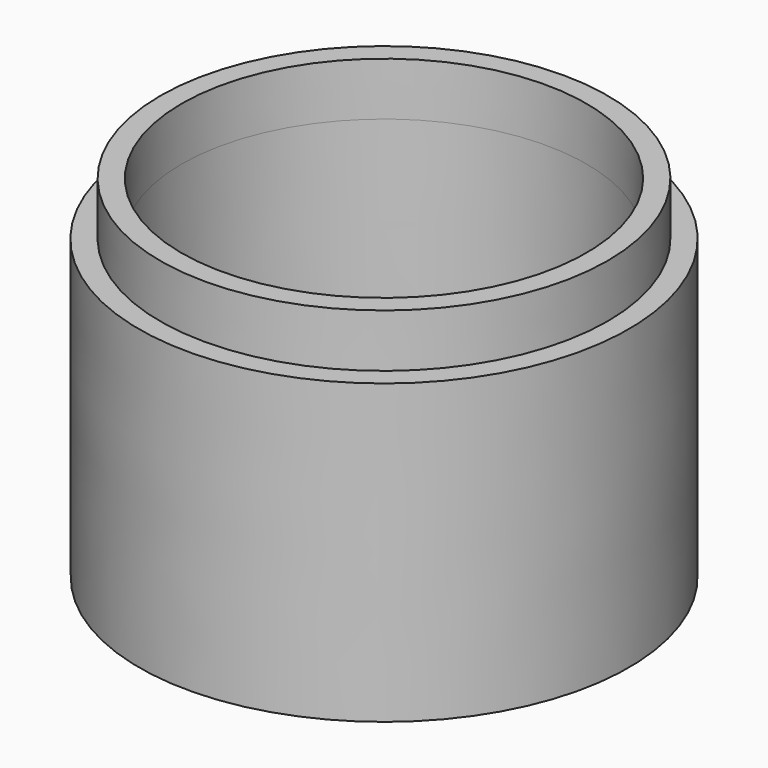
from build123d import *


with BuildPart() as f1:
    # F0 (on Front) → F1 (revolve)
    with BuildSketch(Plane.XZ):
        Polygon((-20.7999995315, 26.2421633642), (-20.7999995315, 21.244951152), (-22.7950242532, 21.2421633642), (-22.7671931058, -6.7578366358), (0.2328019897, -6.736594764), (0.2314215907, -3.7544989489), (-14.966850283, -3.7578366358), (-14.9703099348, 0), (-18.7703107451, 0), (-18.8000003844, 21.2467982709), (-18.8000003844, 26.2421633642), align=None)
    revolve(axis=Axis((0.2321117902, 0, -5.2455468564), (0.0004628955, 0, -0.9999998929)))


solid = f1.part
